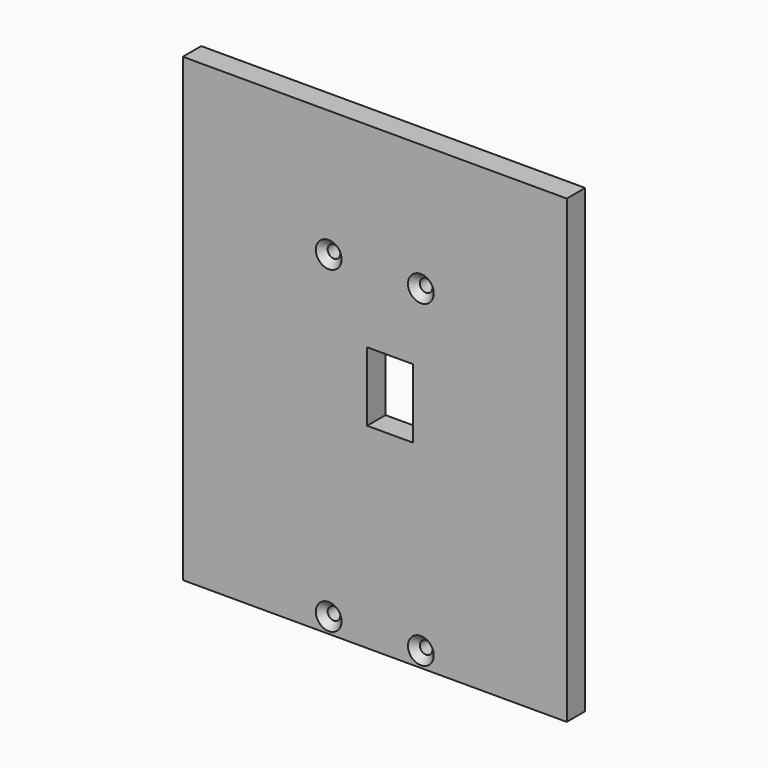
from build123d import *

# Parameters (mm, degrees)
F0_W           = 100
F0_H           = 120
F0_W_2         = 12
F0_H_2         = 18
F1_DEPTH       = 3
F2_SIZE        = 5.99999
F4_D           = 3.3
F4_CSINK_D     = 6.72
F4_CSINK_ANGLE = 90


# Not quite as in the source:
# - a fillet or chamfer is up to 0.001 mm smaller than in the source, because OpenCascade refuses the exact size


with BuildPart() as f1:
    # F0 (on Front) → F1 (new body, symmetric)
    with BuildSketch(Plane.XZ):
        Rectangle(F0_W, F0_H)
        with Locations((4, 0)):
            Rectangle(F0_W_2, F0_H_2, mode=Mode.SUBTRACT)
    extrude(amount=F1_DEPTH, both=True)

    # F2 (size 6 in the source; OpenCascade refuses exactly that, so slightly less here)
    f2_edges = [f1.edges().sort_by_distance(p)[0] for p in [
        (10, 3, 0),
    ]]
    chamfer(f2_edges, length=F2_SIZE)

    # F4 (through all)
    with Locations(Plane.XZ.offset(3)):
        with Locations((-12, 27), (12, 27), (12, -56), (-12, -56)):
            CounterSinkHole(F4_D / 2, F4_CSINK_D / 2, counter_sink_angle=F4_CSINK_ANGLE)


solid = f1.part
